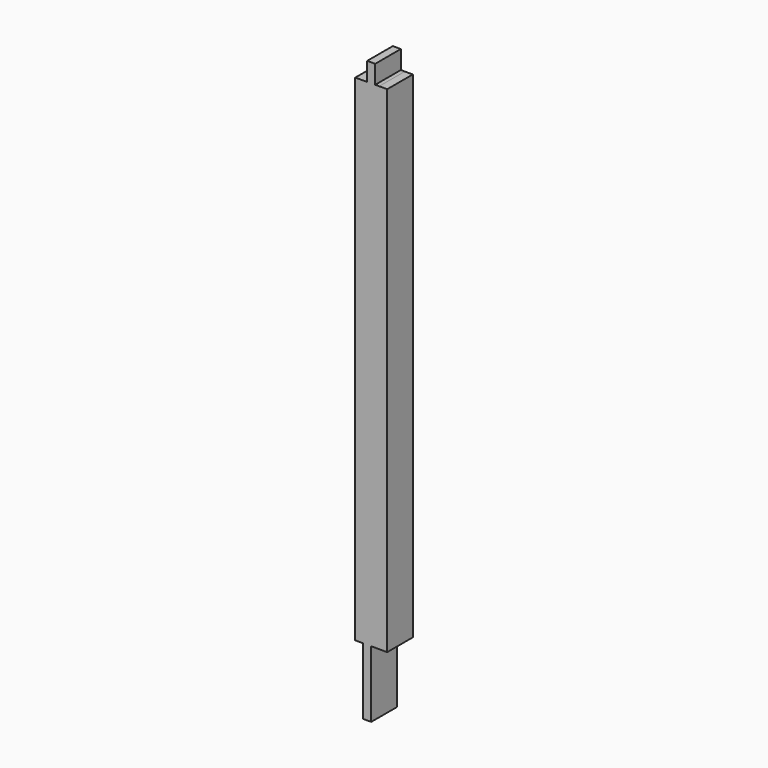
from build123d import *

# Parameters (mm, degrees)
F1_DEPTH = 76.2
F2_W     = 38.1
F2_H     = 152.4
F3_DEPTH = 317.5


# Not quite as in the source:
# - a feature names something its author has since deleted; it is built from what else it names


with BuildPart() as f1:
    # F0 (on Front) → F1 (new body, symmetric)
    with BuildSketch(Plane.XZ):
        Polygon((-19.05, 1136.65), (-76.2, 1136.1958463669), (-76.2, -1225.0958463669), (76.2, -1225.0958463669), (76.2, 1137.1041536331), (38.1, 1137.1041536331), (19.05, 1136.9527690887), (19.05, 1136.65), align=None)
        Polygon((19.05, 1136.9527690887), (-19.05, 1136.65), (19.05, 1136.65), align=None)
        Polygon((19.05, 1225.0958463669), (-19.05, 1225.0958463669), (-19.05, 1136.65), (19.05, 1136.9527690887), align=None)
    extrude(amount=F1_DEPTH, both=True)

    # F2 (on face) → F3 (join)
    with BuildSketch(Plane(origin=(0, 0, -1225.0958463669), x_dir=(1, 0, 0), z_dir=(0, 0, -1))):
        with Locations((-19.05, 0)):
            Rectangle(F2_W, F2_H)
    extrude(amount=F3_DEPTH)


solid = f1.part
